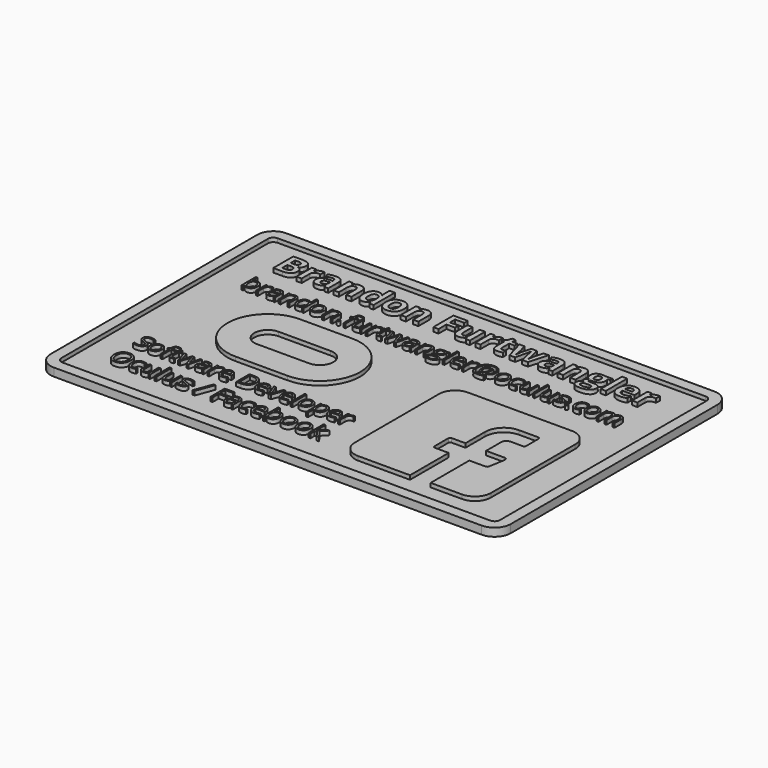
from build123d import *

# Parameters (mm, degrees)
F7_DEPTH     = 0.75
F6_TEXT_SIZE = 4.6465196479
F4_TEXT_SIZE = 4.3980640664
F3_TEXT_SIZE = 6.5258557902
F5_TEXT_SIZE = 4.3243243243
F8_DEPTH     = 1.5


# Not quite as in the source:
# - Text() gives the source's letters only with a copy of the font that has no kerning and outlines rounded to 1/6400 em; it was checked with that copy


with BuildPart() as f7:
    # F0 (on Top) → F7 (new body)
    with BuildSketch(Plane.XY):
        with BuildLine():
            Line((39.75, 23.1077305627), (-39.75, 23.1077305627))
            ThreePointArc((-39.75, 23.1077305627), (-40.4571067812, 22.8148373439), (-40.75, 22.1077305627))
            Line((-40.75, 22.1077305627), (-40.75, -25.8922694373))
            ThreePointArc((-40.75, -25.8922694373), (-40.4571067812, -26.5993762185), (-39.75, -26.8922694373))
            Line((-39.75, -26.8922694373), (39.75, -26.8922694373))
            ThreePointArc((39.75, -26.8922694373), (40.4571067812, -26.5993762185), (40.75, -25.8922694373))
            Line((40.75, -25.8922694373), (40.75, 22.1077305627))
            ThreePointArc((40.75, 22.1077305627), (40.4571067812, 22.8148373439), (39.75, 23.1077305627))
        make_face()
    extrude(amount=F7_DEPTH)

    # F0 (on Top) + F1 (on Top) + F2 (on Top) + F6 (on Top) + F4 (on Top) + F3 (on Top) + F5 (on Top) → F8 (join)
    with BuildSketch(Plane.XY):
        with BuildLine():
            Line((39.75, 25.1077305627), (-39.75, 25.1077305627))
            ThreePointArc((-39.75, 25.1077305627), (-41.8713203436, 24.2290509062), (-42.75, 22.1077305627))
            Line((-42.75, 22.1077305627), (-42.75, -25.8922694373))
            ThreePointArc((-42.75, -25.8922694373), (-41.8713203436, -28.0135897809), (-39.75, -28.8922694373))
            Line((-39.75, -28.8922694373), (39.75, -28.8922694373))
            ThreePointArc((39.75, -28.8922694373), (41.8713203436, -28.0135897809), (42.75, -25.8922694373))
            Line((42.75, -25.8922694373), (42.75, 22.1077305627))
            ThreePointArc((42.75, 22.1077305627), (41.8713203436, 24.2290509062), (39.75, 25.1077305627))
        make_face()
        with BuildLine():
            ThreePointArc((-40.75, 22.1077305627), (-40.4571067812, 22.8148373439), (-39.75, 23.1077305627))
            Line((-39.75, 23.1077305627), (39.75, 23.1077305627))
            ThreePointArc((39.75, 23.1077305627), (40.4571067812, 22.8148373439), (40.75, 22.1077305627))
            Line((40.75, 22.1077305627), (40.75, -25.8922694373))
            ThreePointArc((40.75, -25.8922694373), (40.4571067812, -26.5993762185), (39.75, -26.8922694373))
            Line((39.75, -26.8922694373), (-39.75, -26.8922694373))
            ThreePointArc((-39.75, -26.8922694373), (-40.4571067812, -26.5993762185), (-40.75, -25.8922694373))
            Line((-40.75, -25.8922694373), (-40.75, 22.1077305627))
        make_face(mode=Mode.SUBTRACT)
    with BuildSketch(Plane.XY):
        with BuildLine():
            Line((31.4093656167, 2.5085634552), (12.0937996283, 2.5085634552))
            ThreePointArc((12.0937996283, 2.5085634552), (9.9724792848, 1.6298837988), (9.0937996283, -0.4914365448))
            Line((9.0937996283, -0.4914365448), (9.0937996283, -20.0372585356))
            ThreePointArc((9.0937996283, -20.0372585356), (9.9724792848, -22.1585788792), (12.0937996283, -23.0372585356))
            Line((12.0937996283, -23.0372585356), (21.7515826225, -23.0372585356))
            Line((21.7515826225, -23.0372585356), (21.7515826225, -14.0581438318))
            Line((21.7515826225, -14.0581438318), (19.1341364264, -14.0581438318))
            ThreePointArc((19.1341364264, -14.0581438318), (18.9220043921, -13.9702758661), (18.8341364264, -13.7581438318))
            Line((18.8341364264, -13.7581438318), (18.8341364264, -10.45761399))
            ThreePointArc((18.8341364264, -10.45761399), (18.9220043921, -10.2454819557), (19.1341364264, -10.15761399))
            Line((19.1341364264, -10.15761399), (21.7515826225, -10.15761399))
            Line((21.7515826225, -10.15761399), (21.7515826225, -5.6088223439))
            ThreePointArc((21.7515826225, -5.6088223439), (22.7767088884, -3.1339486097), (25.2515826225, -2.1088223439))
            Line((25.2515826225, -2.1088223439), (28.8716940053, -2.1088223439))
            ThreePointArc((28.8716940053, -2.1088223439), (29.0838260397, -2.1966903095), (29.1716940053, -2.4088223439))
            Line((29.1716940053, -2.4088223439), (29.1716940053, -5.3830801574))
            ThreePointArc((29.1716940053, -5.3830801574), (29.0838260397, -5.5952121918), (28.8716940053, -5.6830801574))
            Line((28.8716940053, -5.6830801574), (26.584375026, -5.6830801574))
            ThreePointArc((26.584375026, -5.6830801574), (25.8772682448, -5.9759733762), (25.584375026, -6.6830801574))
            Line((25.584375026, -6.6830801574), (25.584375026, -10.15761399))
            Line((25.584375026, -10.15761399), (28.9974417876, -10.15761399))
            ThreePointArc((28.9974417876, -10.15761399), (29.3797737985, -10.3353994134), (29.4902135757, -10.7423250564))
            Line((29.4902135757, -10.7423250564), (28.9773130896, -13.7259126849))
            ThreePointArc((28.9773130896, -13.7259126849), (28.8408673204, -13.9640094406), (28.5830956591, -14.0581438318))
            Line((28.5830956591, -14.0581438318), (25.584375026, -14.0581438318))
            Line((25.584375026, -14.0581438318), (25.584375026, -23.0372585356))
            Line((25.584375026, -23.0372585356), (31.4093656167, -23.0372585356))
            ThreePointArc((31.4093656167, -23.0372585356), (33.5306859603, -22.1585788792), (34.4093656167, -20.0372585356))
            Line((34.4093656167, -20.0372585356), (34.4093656167, -0.4914365448))
            ThreePointArc((34.4093656167, -0.4914365448), (33.5306859603, 1.6298837988), (31.4093656167, 2.5085634552))
        make_face()
    with BuildSketch(Plane.XY):
        with BuildLine():
            ThreePointArc((-21.3126111776, 5.2594595402), (-28.8126111776, -2.2405404598), (-21.3126111776, -9.7405404598))
            Line((-21.3126111776, -9.7405404598), (-11.6418842226, -9.7405404598))
            ThreePointArc((-11.6418842226, -9.7405404598), (-4.1418842226, -2.2405404598), (-11.6418842226, 5.2594595402))
            Line((-11.6418842226, 5.2594595402), (-21.3126111776, 5.2594595402))
        make_face()
        with BuildLine():
            Line((-11.6303116083, -4.7405404598), (-21.3115867227, -4.7405404598))
            ThreePointArc((-21.3115867227, -4.7405404598), (-23.8115867227, -2.2405404598), (-21.3115867227, 0.2594595402))
            Line((-21.3115867227, 0.2594595402), (-11.6303116083, 0.2594595402))
            ThreePointArc((-11.6303116083, 0.2594595402), (-9.1303116083, -2.2405404598), (-11.6303116083, -4.7405404598))
        make_face(mode=Mode.SUBTRACT)
    with BuildSketch(Plane.XY):
        with Locations((-35.75, -21.8922694373)):
            Text('Oculus / Facebook', F6_TEXT_SIZE, font='Open Sans', text_align=(TextAlign.LEFT, TextAlign.BOTTOM))
    with BuildSketch(Plane.XY):
        with Locations((-35, 8.2633425926)):
            Text('brandon.furtwangler@oculus.com', F4_TEXT_SIZE, font='Open Sans', text_align=(TextAlign.LEFT, TextAlign.BOTTOM))
    with BuildSketch(Plane.XY):
        with Locations((-35, 15.4091143937)):
            Text('Brandon Furtwangler', F3_TEXT_SIZE, font='Open Sans', font_style=FontStyle.BOLD, text_align=(TextAlign.LEFT, TextAlign.BOTTOM))
    with BuildSketch(Plane.XY):
        with Locations((-35.75, -15.8922694373)):
            Text('Software Developer', F5_TEXT_SIZE, font='Open Sans', text_align=(TextAlign.LEFT, TextAlign.BOTTOM))
    extrude(amount=F8_DEPTH)


solid = f7.part
